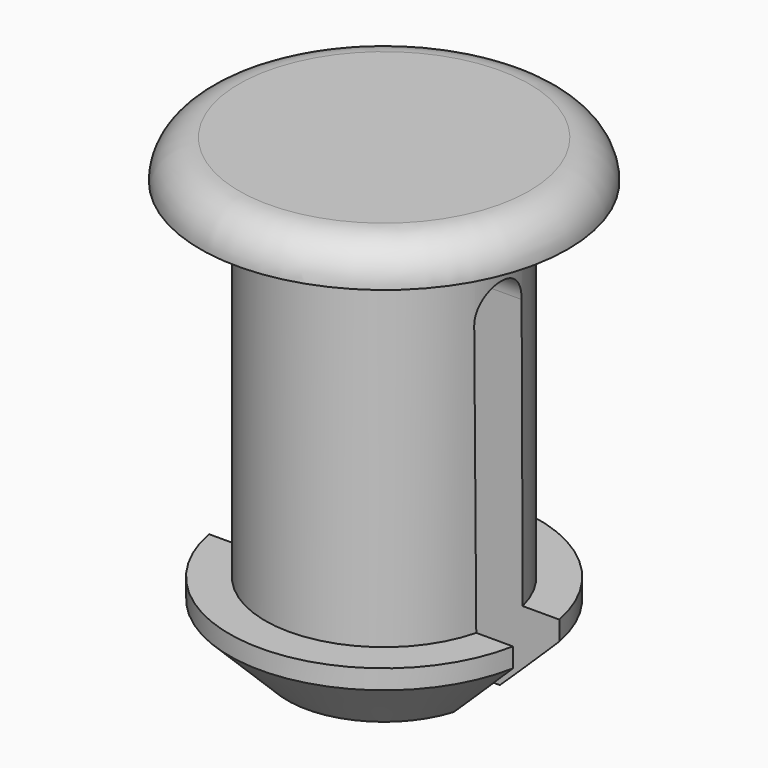
from build123d import *

# Parameters (mm, degrees)
F0_R           = 3.075
F1_DEPTH       = 9
F2_R           = 4.75
F2_R_2         = 3.075
F3_DEPTH       = 1
F4_R           = 0.99999
F5_R           = 4
F5_R_2         = 3.075
F6_DEPTH       = 2
F7_SIZE        = 1.5
F8_R           = 1.5
F9_DEPTH       = 9.5
F11_DEPTH      = 25
F11_DEPTH_BACK = 25


# Not quite as in the source:
# - a fillet or chamfer is up to 0.001 mm smaller than in the source, because OpenCascade refuses the exact size


with BuildPart() as f1:
    # F0 (on Top) → F1 (new body)
    with BuildSketch(Plane.XY):
        Circle(F0_R)
    extrude(amount=F1_DEPTH)

    # F2 (on face) → F3 (join)
    with BuildSketch(Plane.XY.offset(9)):
        Circle(F2_R)
        Circle(F2_R_2, mode=Mode.SUBTRACT)
        Circle(F2_R_2)
    extrude(amount=F3_DEPTH)

    # F4 (radius 1 in the source; OpenCascade refuses exactly that, so slightly less here)
    f4_edges = [f1.edges().sort_by_distance(p)[0] for p in [
        (-4.75, 0, 10),
    ]]
    fillet(f4_edges, radius=F4_R)

    # F5 (on face) → F6 (join)
    with BuildSketch(Plane(origin=(0, 0, 0), x_dir=(1, 0, 0), z_dir=(0, 0, -1))):
        Circle(F5_R)
        Circle(F5_R_2, mode=Mode.SUBTRACT)
        Circle(F5_R_2)
    extrude(amount=F6_DEPTH)

    # F7
    f7_edges = [f1.edges().sort_by_distance(p)[0] for p in [
        (-4, 0, -2),
    ]]
    chamfer(f7_edges, length=F7_SIZE)

    # F8 (on face) → F9 (cut)
    with BuildSketch(Plane(origin=(0, 0, -2), x_dir=(1, 0, 0), z_dir=(0, 0, -1))):
        Circle(F8_R)
    extrude(amount=-F9_DEPTH, mode=Mode.SUBTRACT)

    # F10 (on Right) → F11 (cut, two sides)
    with BuildSketch(Plane.YZ) as f11_sk:
        with BuildLine():
            Line((-0.7, -7), (0.8, -7))
            Line((0.8, -7), (0.7, 7))
            ThreePointArc((0.7, 7), (-0.05, 7.7553762753), (-0.8, 7))
            Line((-0.8, 7), (-0.7, -7))
        make_face()
    extrude(amount=F11_DEPTH, mode=Mode.SUBTRACT)
    extrude(f11_sk.sketch, amount=-F11_DEPTH_BACK, mode=Mode.SUBTRACT)


solid = f1.part
